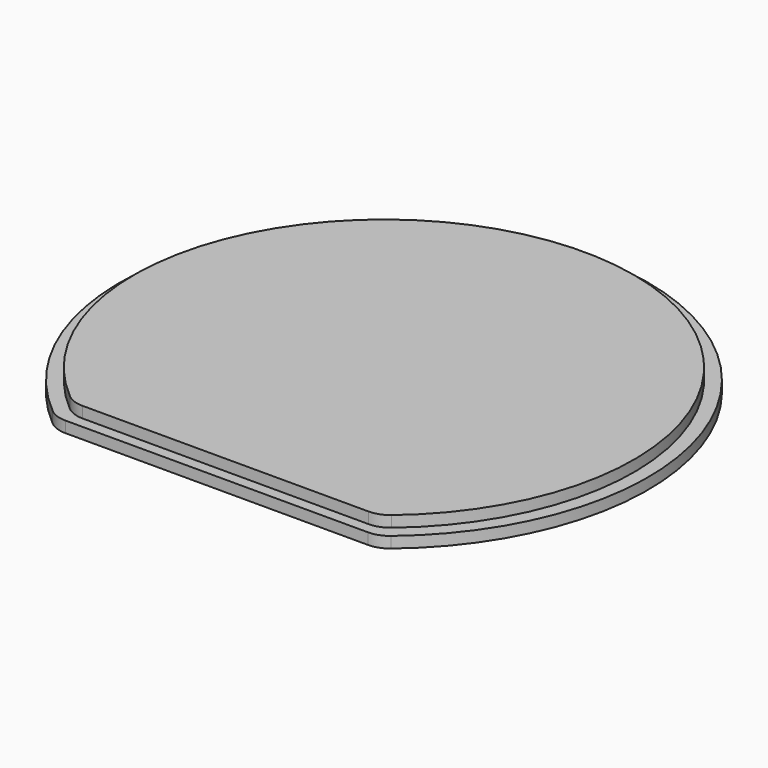
from build123d import *

# Parameters (mm, degrees)
F1_DEPTH = 2
F3_DEPTH = 2
F4_R     = 5


with BuildPart() as f1:
    # F0 (on Top) → F1 (new body)
    with BuildSketch(Plane.XY):
        with BuildLine():
            Line((-27.5, -35.6195171219), (27.5, -35.6195171219))
            ThreePointArc((27.5, -35.6195171219), (0, 45), (-27.5, -35.6195171219))
        make_face()
    extrude(amount=F1_DEPTH)

    # F2 (on face) → F3 (join)
    with BuildSketch(Plane(origin=(0, 0, 0), x_dir=(1, 0, 0), z_dir=(0, 0, -1))):
        with BuildLine():
            Line((29.0003781271, 37.6195171219), (-29.0003781271, 37.6195171219))
            ThreePointArc((-29.0003781271, 37.6195171219), (0, -47.5), (29.0003781271, 37.6195171219))
        make_face()
        with BuildLine():
            Line((-27.5, 35.6195171219), (27.5, 35.6195171219))
            ThreePointArc((27.5, 35.6195171219), (0, -45), (-27.5, 35.6195171219))
        make_face(mode=Mode.SUBTRACT)
        with BuildLine():
            ThreePointArc((-27.5, 35.6195171219), (0, -45), (27.5, 35.6195171219))
            Line((27.5, 35.6195171219), (-27.5, 35.6195171219))
        make_face()
    extrude(amount=F3_DEPTH)

    # F4
    f4_edges = [f1.edges().sort_by_distance(p)[0] for p in [
        (27.5, -35.619517, 1),
        (-29.000378, -37.619517, -1),
        (29.000378, -37.619517, -1),
        (-27.5, -35.619517, 1),
    ]]
    fillet(f4_edges, radius=F4_R)


solid = f1.part
